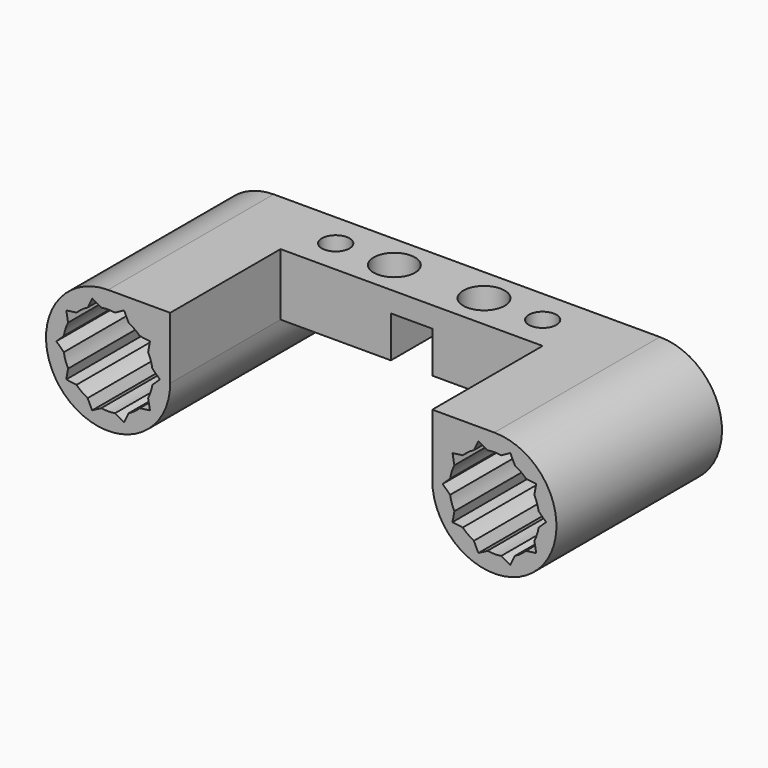
from build123d import *

# Parameters (mm, degrees)
F0_R            = 6.5
F1_DEPTH        = 25
F2_W            = 19
F2_H            = 9
F3_DEPTH        = 15
F4_R            = 2
F5_DEPTH        = 18.001
F7_DEPTH        = 25.001
F7_COPIES_COUNT = 10
F9_DEPTH        = 4
F10_DEPTH       = 5
F12_D           = 6
F12_DEPTH       = 4
F12_TIP         = 1.8025818571
F13_W           = 3
F13_H           = 6
F14_DEPTH       = 30.001


# Not quite as in the source:
# - a pattern or mirror of a feature is missing from the dataset's text; its kind, count and spacing are read off the source's solid


with BuildPart() as f1:
    # F0 (on Front) → F1 (new body)
    with BuildSketch(Plane.XZ):
        with BuildLine():
            Line((-19, 0), (0, 0))
            Line((0, 0), (0, 9))
            Line((0, 9), (-28, 9))
            ThreePointArc((-28, 9), (-21.6360389693, 6.3639610307), (-19, 0))
        make_face()
        with BuildLine():
            ThreePointArc((-28, 9), (-34.3639610307, -6.3639610307), (-19, 0))
            ThreePointArc((-19, 0), (-21.6360389693, 6.3639610307), (-28, 9))
        make_face()
        with Locations((-28, 0)):
            Circle(F0_R, mode=Mode.SUBTRACT)
    extrude(amount=F1_DEPTH)

    # F2 (on face) → F3 (cut)
    with BuildSketch(Plane.XZ.offset(25)):
        with Locations((-9.5, 4.5)):
            Rectangle(F2_W, F2_H)
    extrude(amount=-F3_DEPTH, mode=Mode.SUBTRACT)

    # F4 (on face) → F5 (cut, through all)
    with BuildSketch(Plane.XY.offset(9)):
        with Locations((-15, -5)):
            Circle(F4_R)
    extrude(amount=-F5_DEPTH, mode=Mode.SUBTRACT)

    # F6 (on face) → F7 (cut, through all)
    with BuildSketch(Plane.XZ.offset(25)):
        with BuildLine():
            Line((-21.5833333333, -1.0374916332), (-20.5, 0))
            Line((-20.5, 0), (-21.5833333333, 1.0374916332))
            ThreePointArc((-21.5833333333, 1.0374916332), (-21.5, 0), (-21.5833333333, -1.0374916332))
        make_face()
    f7 = extrude(amount=-F7_DEPTH, mode=Mode.SUBTRACT)

    # F7_copies: F7 ×10 about axis
    f7_copies_axis = Axis((-28, 0, 0), (0, 1, 0))
    for i in range(1, F7_COPIES_COUNT):
        add(f7.rotate(f7_copies_axis, i * 360 / F7_COPIES_COUNT), mode=Mode.SUBTRACT)

    # F8 (on face) → F9 (cut)
    with BuildSketch(Plane(origin=(0, 0, 0), x_dir=(1, 0, 0), z_dir=(0, 0, -1))):
        with BuildLine():
            ThreePointArc((-13.1250001976, 1.7524046217), (-11.7524047929, 3.1249999012), (-11.25, 5))
            ThreePointArc((-11.25, 5), (-11.7524048104, 6.8750001292), (-13.1250002583, 8.2475954133))
            ThreePointArc((-13.1250002583, 8.2475954133), (-15.0000000004, 8.75), (-16.8749997424, 8.2475954129))
            ThreePointArc((-16.8749997424, 8.2475954129), (-18.2475951898, 6.8750001288), (-18.75, 5))
            ThreePointArc((-18.75, 5), (-18.2475951898, 3.1249998712), (-16.8749997424, 1.7524045871))
            ThreePointArc((-16.8749997424, 1.7524045871), (-14.9999999654, 1.25), (-13.1250001976, 1.7524046217))
        make_face()
        with BuildLine():
            Line((-11.25, 2.8349364905), (-11.25, 5))
            ThreePointArc((-11.25, 5), (-11.7524047929, 3.1249999012), (-13.1250001976, 1.7524046217))
            Line((-13.1250001976, 1.7524046217), (-11.25, 2.8349364905))
        make_face()
        with BuildLine():
            ThreePointArc((-13.1250002583, 8.2475954133), (-11.7524048104, 6.8750001292), (-11.25, 5))
            Line((-11.25, 5), (-11.25, 7.1650635095))
            Line((-11.25, 7.1650635095), (-13.1250002583, 8.2475954133))
        make_face()
        with BuildLine():
            ThreePointArc((-16.8749997424, 8.2475954129), (-15.0000000004, 8.75), (-13.1250002583, 8.2475954133))
            Line((-13.1250002583, 8.2475954133), (-15, 9.3301270189))
            Line((-15, 9.3301270189), (-16.8749997424, 8.2475954129))
        make_face()
        with BuildLine():
            Line((-15, 0.6698729811), (-13.1250001976, 1.7524046217))
            ThreePointArc((-13.1250001976, 1.7524046217), (-14.9999999654, 1.25), (-16.8749997424, 1.7524045871))
            Line((-16.8749997424, 1.7524045871), (-15, 0.6698729811))
        make_face()
        with BuildLine():
            ThreePointArc((-18.75, 5), (-18.2475951898, 6.8750001288), (-16.8749997424, 8.2475954129))
            Line((-16.8749997424, 8.2475954129), (-18.75, 7.1650635095))
            Line((-18.75, 7.1650635095), (-18.75, 5))
        make_face()
        with BuildLine():
            Line((-18.75, 2.8349364905), (-16.8749997424, 1.7524045871))
            ThreePointArc((-16.8749997424, 1.7524045871), (-18.2475951898, 3.1249998712), (-18.75, 5))
            Line((-18.75, 5), (-18.75, 2.8349364905))
        make_face()
    extrude(amount=-F9_DEPTH, mode=Mode.SUBTRACT)

    # F10 (add): a face of the model
    f10_faces = [f1.faces().sort_by_distance(p)[0] for p in [
        (-34.1839610307, -25, -6.1839610307),
    ]]
    extrude(f10_faces, amount=F10_DEPTH)

    # F12
    with Locations(Plane.XY.offset(9)):
        with Locations((-6.5, -5)):
            Hole(F12_D / 2, depth=F12_DEPTH)
            with Locations((0, 0, -(F12_DEPTH + F12_TIP / 2))):  # 118° drill point
                Cone(0, F12_D / 2, F12_TIP, mode=Mode.SUBTRACT)

    # F13 (on face) → F14 (cut, through all)
    with BuildSketch(Plane(origin=(0, 0, 0), x_dir=(-1, 0, 0), z_dir=(0, 1, 0))):
        with Locations((1.5, 3)):
            Rectangle(F13_W, F13_H)
    extrude(amount=-F14_DEPTH, mode=Mode.SUBTRACT)

    # F15: F1 across plane


with BuildPart() as f1_1:
    add(f1.part)
    add(f1.part.mirror(Plane.YZ))


solid = f1_1.part
